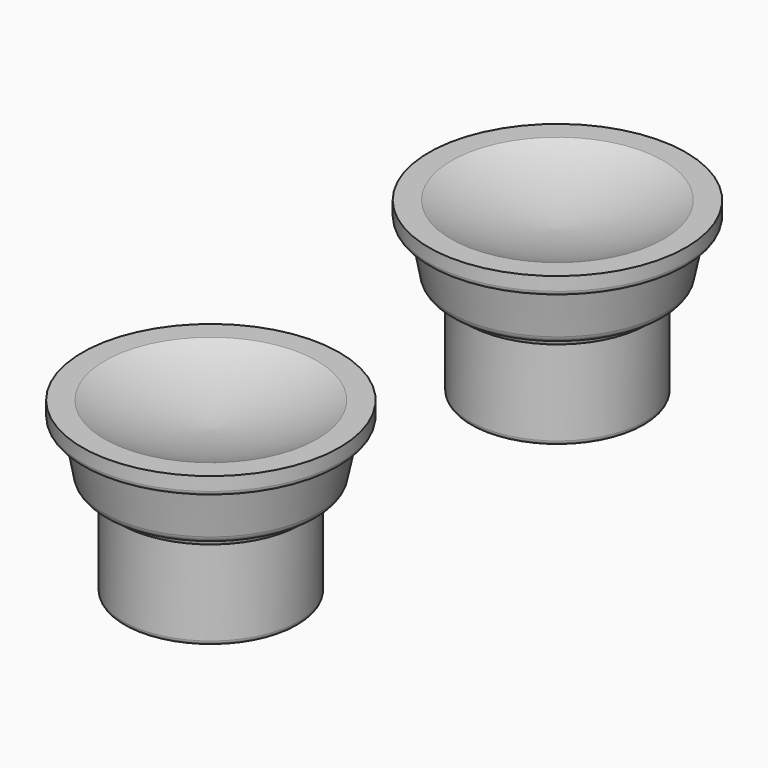
from build123d import *

# Parameters (mm, degrees)
F2_R = 1
F3_R = 2
F4_R = 1
F5_R = 1
F6_R = 0.99999
F7_R = 1


# Not quite as in the source:
# - a fillet or chamfer is up to 0.001 mm smaller than in the source, because OpenCascade refuses the exact size


with BuildPart() as f1:
    # F0 (on Front) → F1 (revolve)
    with BuildSketch(Plane.XZ):
        with BuildLine():
            Line((0, 32.356467098), (0, 0))
            Line((0, 0), (19.5, 0))
            Line((19.5, 0), (19.5, 20))
            Line((19.5, 20), (20.5, 20))
            Line((20.5, 20), (20.5, 22))
            Line((20.5, 22), (23.5, 22))
            Line((23.5, 22), (25.9, 34))
            Line((25.9, 34), (28.6, 34))
            Line((28.6, 34), (28.6, 38))
            Line((28.6, 38), (23.6, 38))
            add(Edge.make_bspline(
                [(23.6, 38), (18.1674417108, 35.3825725615), (8.929848671, 32.6750017703), (0, 32.356467098)],
                knots=[0, 0, 0, 0, 24.265396424, 24.265396424, 24.265396424, 24.265396424], degree=3))
        make_face()
    revolve(axis=Axis((0, 0, 16.178233549), (0, 0, 1)))

    # F2
    f2_edges = [f1.edges().sort_by_distance(p)[0] for p in [
        (-19.5, 0, 0),
    ]]
    fillet(f2_edges, radius=F2_R)

    # F3
    f3_edges = [f1.edges().sort_by_distance(p)[0] for p in [
        (-23.5, 0, 22),
    ]]
    fillet(f3_edges, radius=F3_R)

    # F4
    f4_edges = [f1.edges().sort_by_distance(p)[0] for p in [
        (-28.6, 0, 34),
    ]]
    fillet(f4_edges, radius=F4_R)

    # F5
    f5_edges = [f1.edges().sort_by_distance(p)[0] for p in [
        (-25.9, 0, 34),
    ]]
    fillet(f5_edges, radius=F5_R)

    # F6 (radius 1 in the source; OpenCascade refuses exactly that, so slightly less here)
    f6_edges = [f1.edges().sort_by_distance(p)[0] for p in [
        (-20.5, 0, 20),
    ]]
    fillet(f6_edges, radius=F6_R)

    # F7
    f7_edges = [f1.edges().sort_by_distance(p)[0] for p in [
        (-20.5, 0, 22),
    ]]
    fillet(f7_edges, radius=F7_R)


with BuildPart() as f8_1:
    # F8: copy of F1
    add(f1.part.moved(Location((0, 96.3, 0))))


solid = Compound([f1.part, f8_1.part])
